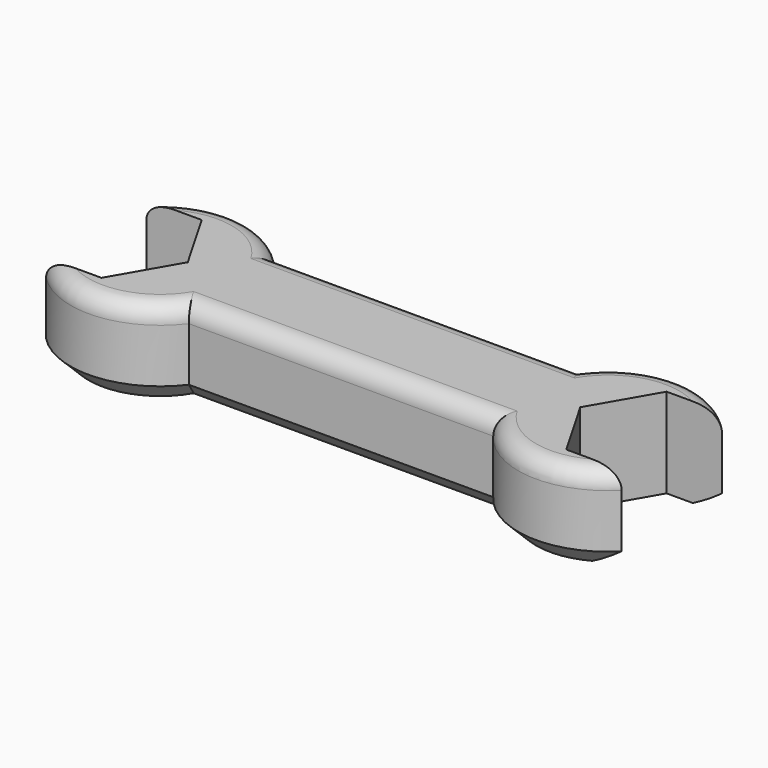
from build123d import *

# Parameters (mm, degrees)
F1_DEPTH = 6.35
F3_DEPTH = 12.701
F6_R     = 2.54
F7_SIZE  = 2.54


with BuildPart() as f1:
    # F0 (on Top) → F1 (new body, symmetric)
    with BuildSketch(Plane.XY):
        with BuildLine():
            Line((21.59, 7.62), (-21.59, 7.62))
            ThreePointArc((-21.59, 7.62), (-44.45, 0), (-21.59, -7.62))
            Line((-21.59, -7.62), (21.59, -7.62))
            ThreePointArc((21.59, -7.62), (44.45, 0), (21.59, 7.62))
        make_face()
    extrude(amount=F1_DEPTH, both=True)

    # F4: F3 across plane


with BuildPart() as f3:
    # F2 (on face) → F3 (new body, through all)
    with BuildSketch(Plane.XY.offset(6.35)):
        Polygon((-43.2326438931, 8.89), (-48.3652877862, 0), (-43.2326438931, -8.89), (-32.9673561069, -8.89), (-27.8347122138, 0), (-32.9673561069, 8.89), align=None)
    extrude(amount=-F3_DEPTH)


with BuildPart() as f1_1:
    add(f1.part)
    add(f3.part.mirror(Plane.YZ), mode=Mode.SUBTRACT)

    # F5: cut F3
    add(f3.part, mode=Mode.SUBTRACT)

    # F6
    f6_edges = [f1_1.edges().sort_by_distance(p)[0] for p in [
        (-30.913065, -12.672393, 6.35),
        (0, -7.62, 6.35),
        (30.913065, -12.672393, 6.35),
        (30.913065, 12.672393, 6.35),
        (0, 7.62, 6.35),
        (-30.913065, 12.672393, 6.35),
    ]]
    fillet(f6_edges, radius=F6_R)

    # F7
    f7_edges = [f1_1.edges().sort_by_distance(p)[0] for p in [
        (-30.913065, 12.672393, -6.35),
        (0, 7.62, -6.35),
        (30.913065, 12.672393, -6.35),
        (30.913065, -12.672393, -6.35),
        (0, -7.62, -6.35),
        (-30.913065, -12.672393, -6.35),
    ]]
    chamfer(f7_edges, length=F7_SIZE)


solid = f1_1.part
